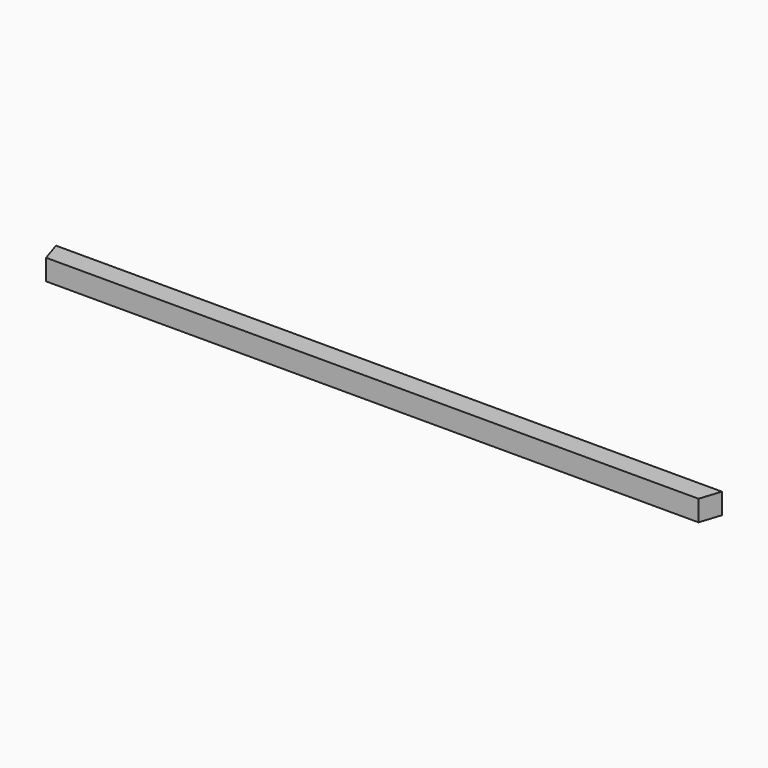
from build123d import *

# Parameters (mm, degrees)
F0_W     = 101.6
F0_H     = 3.175
F1_DEPTH = 3.175
F2_SIZE2 = 1.03161
F2_SIZE  = 3.17499
F3_SIZE2 = 1.03161
F3_SIZE  = 3.17499


# Not quite as in the source:
# - a fillet or chamfer is up to 0.001 mm smaller than in the source, because OpenCascade refuses the exact size


with BuildPart() as f1:
    # F0 (on Front) → F1 (new body)
    with BuildSketch(Plane.XZ):
        with Locations((-38.2536438465, -4.0487329051)):
            Rectangle(F0_W, F0_H)
    extrude(amount=F1_DEPTH)

    # F2 (size 3.175 and 1.0316200355 in the source; OpenCascade refuses exactly that, so slightly less here)
    f2_edges = [f1.edges().sort_by_distance(p)[0] for p in [
        (-89.053644, -3.175, -4.048733),
    ]]
    f2_side = f1.faces().sort_by_distance((-89.053644, -1.5875, -4.048733))[0]
    chamfer(f2_edges, length=F2_SIZE, length2=F2_SIZE2, reference=f2_side)

    # F3 (size 3.175 and 1.0316200355 in the source; OpenCascade refuses exactly that, so slightly less here)
    f3_edges = [f1.edges().sort_by_distance(p)[0] for p in [
        (12.546356, -3.175, -4.048733),
    ]]
    f3_side = f1.faces().sort_by_distance((12.546356, -1.5875, -4.048733))[0]
    chamfer(f3_edges, length=F3_SIZE, length2=F3_SIZE2, reference=f3_side)


solid = f1.part
